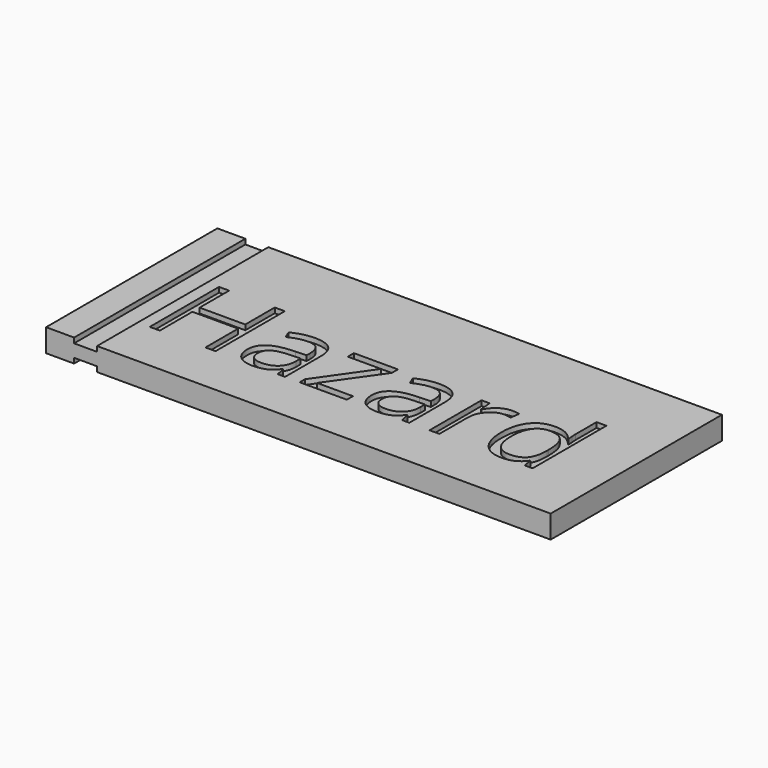
from build123d import *

# Parameters (mm, degrees)
F0_W         = 198
F0_H         = 84
F1_DEPTH     = 9
F2_TEXT_SIZE = 47.6217387209
F3_DEPTH     = 2
F2_W         = 9
F2_H         = 84
F4_DEPTH     = 2
F5_W         = 9
F5_H         = 84
F6_DEPTH     = 2


# Not quite as in the source:
# - Text() gives the source's letters only with a copy of the font that has no kerning and outlines rounded to 1/6400 em; it was checked with that copy


with BuildPart() as f1:
    # F0 (on Top) → F1 (new body)
    with BuildSketch(Plane.XY):
        Rectangle(F0_W, F0_H)
    extrude(amount=F1_DEPTH)

    # F2 (on face) → F3 (cut)
    with BuildSketch(Plane.XY.offset(9)):
        with Locations((-79, -22)):
            Text('Hazard', F2_TEXT_SIZE, font='Open Sans', text_align=(TextAlign.LEFT, TextAlign.BOTTOM))
    extrude(amount=-F3_DEPTH, mode=Mode.SUBTRACT)

    # F2 (on face) → F4 (cut)
    with BuildSketch(Plane.XY.offset(9)):
        with Locations((-83.5, 0)):
            Rectangle(F2_W, F2_H)
    extrude(amount=-F4_DEPTH, mode=Mode.SUBTRACT)

    # F5 (on face) → F6 (cut)
    with BuildSketch(Plane(origin=(0, 0, 0), x_dir=(1, 0, 0), z_dir=(0, 0, -1))):
        with Locations((-83.5, 0)):
            Rectangle(F5_W, F5_H)
    extrude(amount=-F6_DEPTH, mode=Mode.SUBTRACT)


solid = f1.part
